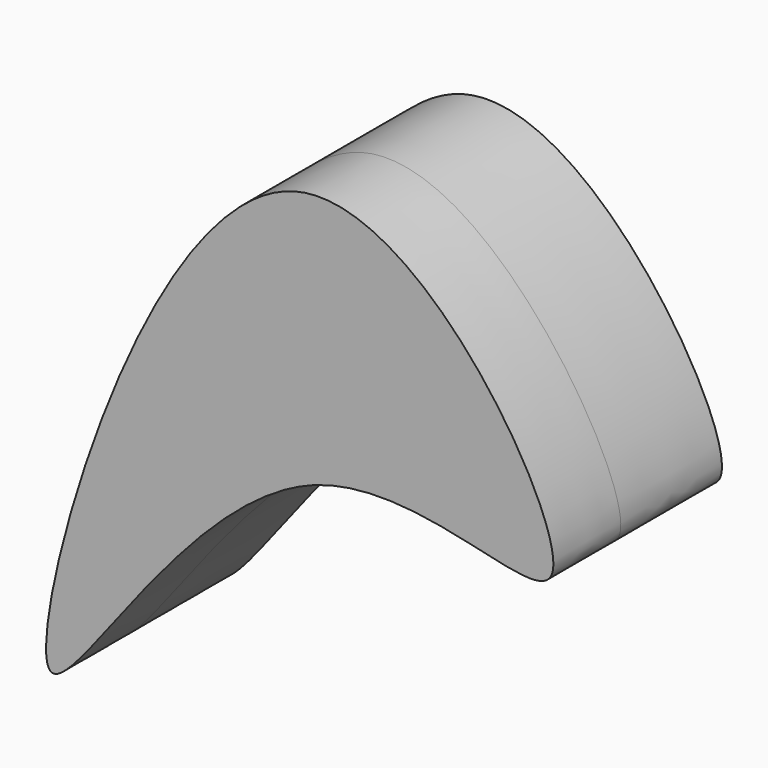
from build123d import *

# Parameters (mm, degrees)
F1_DEPTH = 38.1
F4_W     = 6.5451301634
F4_H     = 14.025259763
F5_DEPTH = 25.4


# Not quite as in the source:
# - the program builds the solid bodies; features that only make, move or delete a surface that nothing else refers to are left out


with BuildPart() as f1:
    # F0 (on Front) → F1 (new body)
    with BuildSketch(Plane.XZ):
        with BuildLine():
            add(Edge.make_bspline(
                [(4.3095196597, 0), (36.5053707041, 11.7644892129), (116.333305535, -41.5678144416), (-17.4601458028, 170.8669328795), (-111.9350192378, -169.009166265), (-35.4037927626, -14.5113988432), (4.3095196597, 0)],
                knots=[0, 0, 0, 0, 0.2003144859, 0.4457556905, 0.7529137605, 1, 1, 1, 1], degree=3))
        make_face()
    extrude(amount=F1_DEPTH)

    # F4 (on face) → F5 (join)
    with BuildSketch(Plane.XZ.offset(38.1)):
        with BuildLine():
            add(Edge.make_bspline(
                [(4.3095196597, 0), (36.5053707041, 11.7644892129), (116.333305535, -41.5678144416), (-17.4601458028, 170.8669328795), (-111.9350192378, -169.009166265), (-35.4037927626, -14.5113988432), (4.3095196597, 0)],
                knots=[0, 0, 0, 0, 0.2003144859, 0.4457556905, 0.7529137605, 1, 1, 1, 1], degree=3))
        make_face()
        Polygon((9.0551180765, 48.0109006166), (9.0551180765, 62.3478330672), (14.6652227268, 62.0361603796), (14.6652227268, 48.0109006166), align=None, mode=Mode.SUBTRACT)
        with Locations((28.2229799777, 55.0235304981)):
            Rectangle(F4_W, F4_H, mode=Mode.SUBTRACT)
        with Locations((28.2229799777, 55.0235304981)):
            Rectangle(F4_W, F4_H)
        Polygon((14.6652227268, 62.0361603796), (9.0551180765, 62.3478330672), (9.0551180765, 48.0109006166), (14.6652227268, 48.0109006166), align=None)
    extrude(amount=F5_DEPTH)


solid = f1.part
